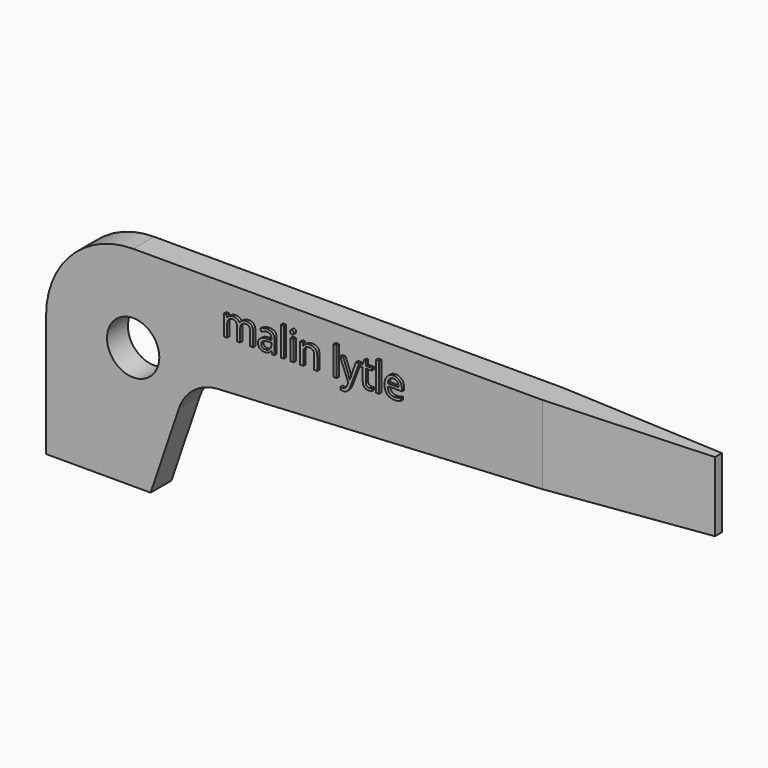
from build123d import *

# Parameters (mm, degrees)
F1_DEPTH     = 2.38125
F2_R         = 2.38125
F3_DEPTH     = 2.38225
F5_DEPTH     = 25.4
F6_TEXT_SIZE = 3.4852225023
F7_DEPTH     = 0.254


# Not quite as in the source:
# - Text() gives the source's letters only with a copy of the font that has no kerning and outlines rounded to 1/6400 em; it was checked with that copy


with BuildPart() as f1:
    # F0 (on Front) → F1 (new body)
    with BuildSketch(Plane.XZ):
        with BuildLine():
            Line((60.325, 12.7), (60.325, 19.05))
            Line((60.325, 19.05), (7.9375, 19.05))
            ThreePointArc((7.9375, 19.05), (2.3248399243, 16.7251600757), (0, 11.1125))
            Line((0, 11.1125), (0, 0))
            Line((0, 0), (9.525, 0))
            Line((9.525, 0), (12.1173647876, 7.6271664624))
            ThreePointArc((12.1173647876, 7.6271664624), (13.4786145605, 9.5135918491), (15.6631963617, 10.3130942181))
            Line((15.6631963617, 10.3130942181), (60.325, 12.7))
        make_face()
    extrude(amount=F1_DEPTH)

    # F2 (on face) → F3 (cut, through all)
    with BuildSketch(Plane.XZ.offset(2.38125)):
        with Locations((7.9375, 11.1125)):
            Circle(F2_R)
    extrude(amount=-F3_DEPTH, mode=Mode.SUBTRACT)

    # F4 (on face) → F5 (cut)
    with BuildSketch(Plane.XY.offset(19.05)):
        Polygon((60.325, -2.38125), (60.325, -1.5875), (45.24375, -2.38125), align=None)
        Polygon((45.24375, 0), (60.325, -0.79375), (60.325, 0), align=None)
    extrude(amount=-F5_DEPTH, mode=Mode.SUBTRACT)

    # F6 (on face) → F7 (join)
    with BuildSketch(Plane.XZ.offset(2.38125)):
        with Locations((16.1178186536, 14.8631362244)):
            Text('malin lytle', F6_TEXT_SIZE, font='Open Sans', text_align=(TextAlign.LEFT, TextAlign.BOTTOM))
    extrude(amount=F7_DEPTH)


solid = f1.part
